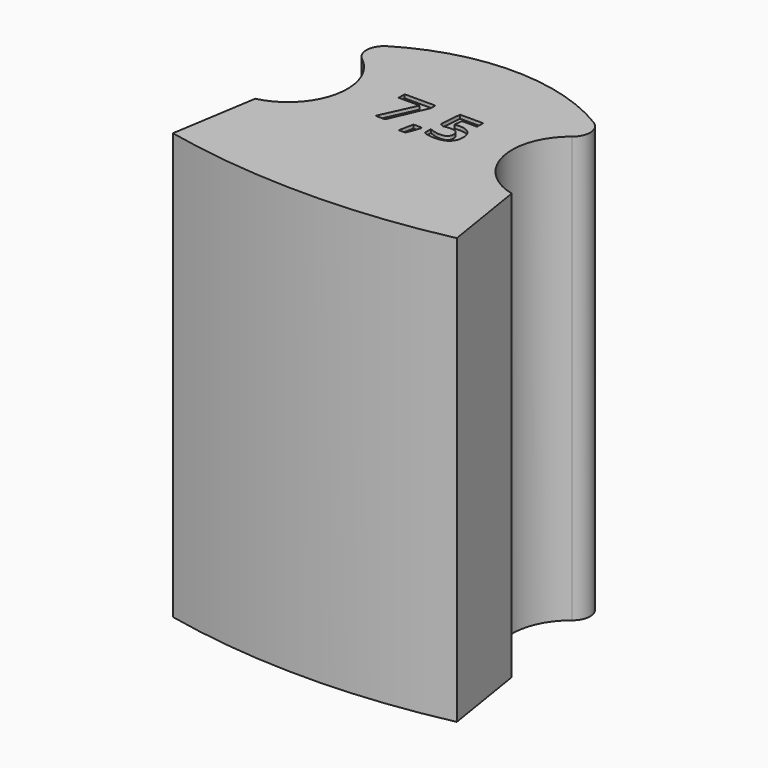
from build123d import *

# Parameters (mm, degrees)
F1_DEPTH     = 120
F2_TEXT_SIZE = 16.856395329
F3_DEPTH     = 1


# Not quite as in the source:
# - Text() gives the source's letters only with a copy of the font that has no kerning and outlines rounded to 1/6400 em; it was checked with that copy


with BuildPart() as f1:
    # F0 (on Top) → F1 (new body)
    with BuildSketch(Plane.XY):
        with BuildLine():
            Line((3.8687128108, 24.1569802165), (0, 0))
            ThreePointArc((0, 0), (40, -4.2812949374), (80, 0))
            Line((80, 0), (76.1312871892, 24.1569802165))
            ThreePointArc((76.1312871892, 24.1569802165), (63.5975554576, 36.8458138953), (69.5972800683, 53.6417728094))
            ThreePointArc((69.5972800683, 53.6417728094), (71.4969098635, 57.8715436357), (69.1043731597, 61.843359684))
            ThreePointArc((69.1043731597, 61.843359684), (40, 70), (10.8956268403, 61.843359684))
            ThreePointArc((10.8956268403, 61.843359684), (8.5030901365, 57.8715436357), (10.4027199317, 53.6417728094))
            ThreePointArc((10.4027199317, 53.6417728094), (16.4024445424, 36.8458138953), (3.8687128108, 24.1569802165))
        make_face()
    extrude(amount=F1_DEPTH)

    # F2 (on face) → F3 (cut)
    with BuildSketch(Plane.XY.offset(120)):
        with Locations((27.7659443276, 34.3472510576)):
            Text('7,5', F2_TEXT_SIZE, font='Open Sans', font_style=FontStyle.BOLD, text_align=(TextAlign.LEFT, TextAlign.BOTTOM))
    extrude(amount=-F3_DEPTH, mode=Mode.SUBTRACT)


solid = f1.part
